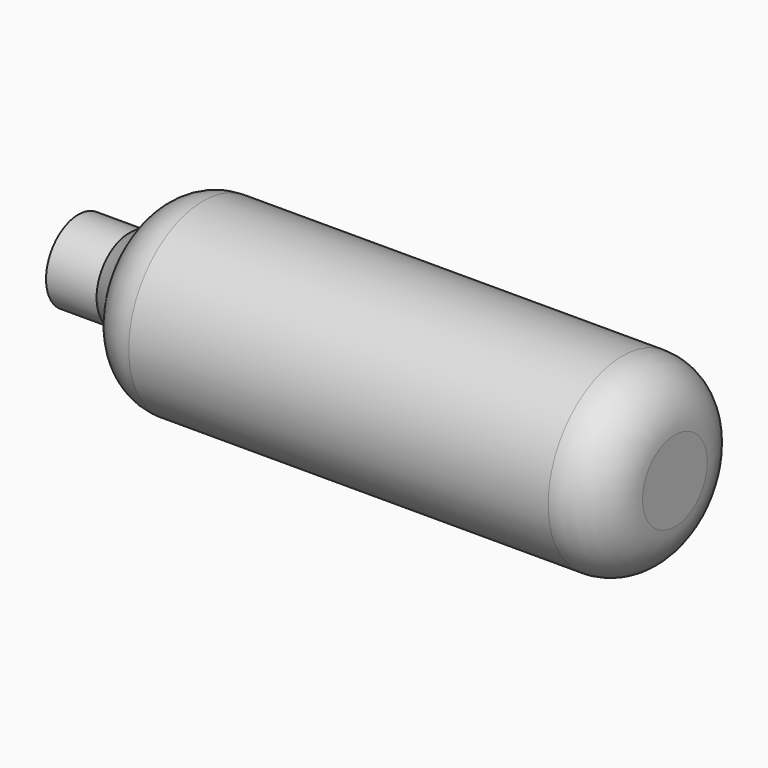
from build123d import *

# Parameters (mm, degrees)
F0_R     = 9
F1_DEPTH = 50.8
F2_R     = 5.08
F3_DEPTH = 7


# Not quite as in the source:
# - a fillet or chamfer that OpenCascade refuses, or shapes differently, is made with other operations: its cross-section is extruded or revolved along the edge and cut away or added


with BuildPart() as f1:
    # F0 (on Right) → F1 (new body)
    with BuildSketch(Plane.YZ):
        Circle(F0_R)
    extrude(amount=F1_DEPTH)

    # F2
    f2_edges = [f1.edges().sort_by_distance(p)[0] for p in [
        (50.8, -9, 0),
        (0, -9, 0),
    ]]
    fillet(f2_edges, radius=F2_R)

    # F3 (add): a face of the model
    f3_faces = [f1.faces().sort_by_distance(p)[0] for p in [
        (0, 0, 0),
    ]]
    extrude(f3_faces, amount=F3_DEPTH)

    # F4: chamfer of 2.54 on 1 edges, made by hand

    # F4_s1 → F4_t2 (revolve)
    with BuildSketch(Plane.XY):
        with BuildLine():
            Line((0.2905300688, 5.6133333333), (-2.1042048969, 3.92))
            Line((-2.1042048969, 3.92), (0, 3.92))
            ThreePointArc((0, 3.92), (0.0794974837, 4.8151952776), (0.2905300688, 5.6133333333))
        make_face()
    revolve(axis=Axis((0, 0, 0), (1, 0, 0)))


solid = f1.part
